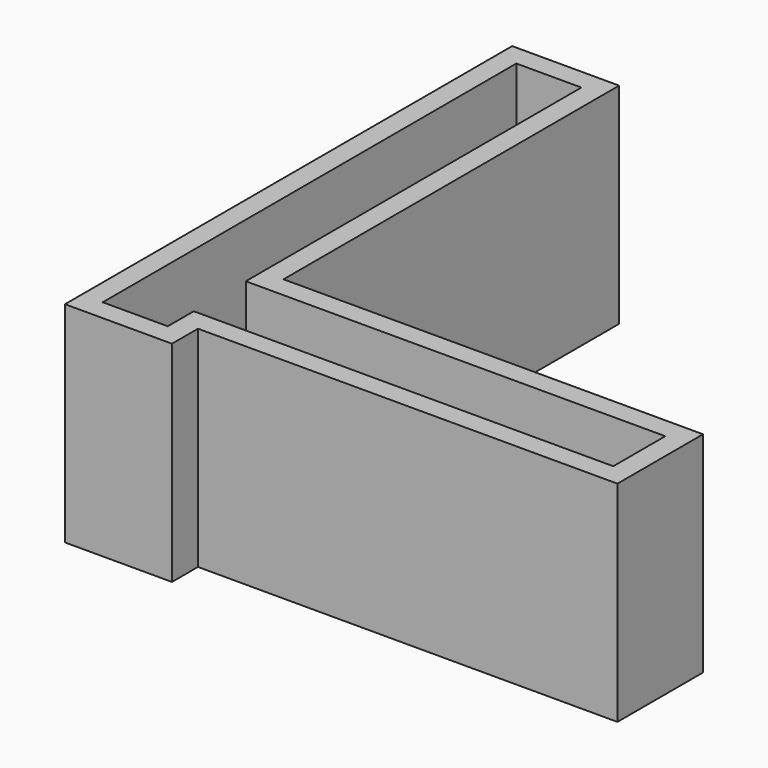
from build123d import *

# Parameters (mm, degrees)
F1_W     = 50.2
F1_H     = 53.3
F2_DEPTH = 20
F3_DEPTH = 14
F4_W     = 40
F4_H     = 40
F4_H_2   = 3.1
F5_DEPTH = 20.001


# Not quite as in the source:
# - a feature of the source that left no trace in its solid (it failed there, or was rolled back) is left out


with BuildPart() as f2:
    # F1 (on Top) → F2 (new body)
    with BuildSketch(Plane.XY):
        with Locations((23.1, 24.65)):
            Rectangle(F1_W, F1_H)
    extrude(amount=-F2_DEPTH)

    # F0 (on Top) → F3 (cut)
    with BuildSketch(Plane.XY):
        Polygon((6.2, 49.3), (0, 49.3), (0, 0), (6.2, 0), (6.2, 3.1), (46.2, 3.1), (46.2, 9.3), (6.2, 9.3), align=None)
    extrude(amount=-F3_DEPTH, mode=Mode.SUBTRACT)

    # F4 (on face) → F5 (cut, through all)
    with BuildSketch(Plane.XY):
        with Locations((28.2, 31.3)):
            Rectangle(F4_W, F4_H)
        with Locations((28.2, -0.45)):
            Rectangle(F4_W, F4_H_2)
    extrude(amount=-F5_DEPTH, mode=Mode.SUBTRACT)


solid = f2.part
